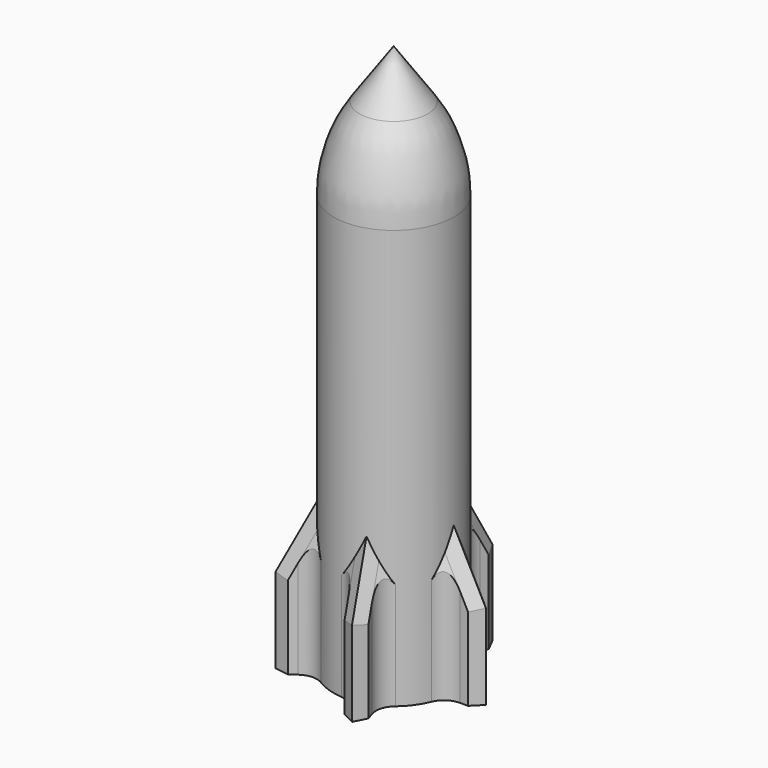
from build123d import *

# Parameters (mm, degrees)
F0_R          = 15.31
F0_R_2        = 11.5
F1_DEPTH      = 101.6
F2_DEPTH      = 25.4
F3_DEPTH      = 25.4
F4_DEPTH      = 25.4
F5_DEPTH      = 25.4
F6_R          = 15.31
F7_DEPTH      = 25.4
F7_TAPER      = 35
F8_T          = 2.54
F10_DEPTH     = 2.54
F11_DEPTH     = 10.668
F12_COUNT     = 5
F14_SIZE      = 2.5399
F15_DEPTH     = 25.4
F16_T1_DEPTH  = 31.2479879022
F16_T3_DEPTH  = 26.3887057153
F16_T5_DEPTH  = 18.1838383234
F16_T7_DEPTH  = 38.4641495789
F17_DEPTH     = 19.304
F18_R         = 36.6377921473
F19_T1_DEPTH  = 6.096
F19_T6_DEPTH  = 35.9639195383
F19_T11_DEPTH = 35.9639195383
F19_T16_DEPTH = 35.9639195383
F19_T21_DEPTH = 35.9639195383
F19_T26_DEPTH = 35.9639195383
F19_T31_DEPTH = 35.9639195383
F19_T36_DEPTH = 35.9639195383
F19_T41_DEPTH = 35.9639195383
F19_T46_DEPTH = 35.9639195383
F19_T51_DEPTH = 35.9639195383


# Not quite as in the source:
# - a fillet or chamfer that OpenCascade refuses, or shapes differently, is made with other operations: its cross-section is extruded or revolved along the edge and cut away or added
# - a fillet or chamfer is up to 0.001 mm smaller than in the source, because OpenCascade refuses the exact size
# - a shell that OpenCascade refuses in one call is made with other operations: the cavity is built on its own and cut out


with BuildPart() as f1:
    # F0 (on Top) → F1 (new body)
    with BuildSketch(Plane.XY):
        Circle(F0_R)
        Circle(F0_R_2, mode=Mode.SUBTRACT)
    extrude(amount=F1_DEPTH)

    # F2 (add): a face of the model
    f2_faces = [f1.faces().sort_by_distance(p)[0] for p in [
        (-14.8769678072, 0, 101.6),
    ]]
    extrude(f2_faces, amount=F2_DEPTH)

    # F3 (cut): a face of the model
    f3_faces = [f1.faces().sort_by_distance(p)[0] for p in [
        (-14.8769678072, 0, 127),
    ]]
    extrude(f3_faces, amount=-F3_DEPTH, mode=Mode.SUBTRACT)

    # F4 (add): a face of the model
    f4_faces = [f1.faces().sort_by_distance(p)[0] for p in [
        (-14.8769678072, 0, 101.6),
    ]]
    extrude(f4_faces, amount=F4_DEPTH)

    # F5 (cut): a face of the model
    f5_faces = [f1.faces().sort_by_distance(p)[0] for p in [
        (-14.8769678072, 0, 127),
    ]]
    extrude(f5_faces, amount=-F5_DEPTH, mode=Mode.SUBTRACT)

    # F6 (on face) → F7 (join)
    with BuildSketch(Plane.XY.offset(101.6)):
        Circle(F6_R)
    extrude(amount=F7_DEPTH, taper=F7_TAPER)

    # F8: shell of thickness 2.54, made by hand


with BuildPart() as f8_core1:
    # F8_t2: copy of F1
    add(f1.part)

    # the walls: a layer under each face that stays
    f8_faces = [f8_core1.faces().sort_by_distance(p)[0] for p in [
        (-15.31, 0, 50.8),
        (-7.655, 0, 112.5324729916),
        (-10.2066666667, -10.2066666667, 0),
        (-11.5, 0, 50.8),
    ]]
    thicken(f8_faces, amount=-F8_T, mode=Mode.SUBTRACT)


with BuildPart() as f1_1:
    add(f1.part)

    # what is left inside the walls is the cavity
    f8_cavity = [f8_core1.part.solids().sort_by_distance(p)[0] for p in [
        (-8.118682, 0, 107.397628),
    ]]
    add(f8_cavity, mode=Mode.SUBTRACT)

    # F9 (on Front) → F10 (join, symmetric)
    with BuildSketch(Plane.XZ):
        Polygon((26.068892777, 0), (12.5377972627, 26.279142328), (12.7, 0), align=None)
    extrude(amount=F10_DEPTH, both=True)

    # F11 (add): a face of the model
    f11_faces = [f1_1.faces().sort_by_distance(p)[0] for p in [
        (-14.7952381942, 0, 0),
    ]]
    extrude(f11_faces, amount=F11_DEPTH)


with BuildPart() as f12_1:
    # F12: instance of F1
    add(f1_1.part.rotate(Axis((0, 0, 0), (0, 0, 1)), 1 * 360 / F12_COUNT))


with BuildPart() as f12_2:
    # F12: instance of F1
    add(f1_1.part.rotate(Axis((0, 0, 0), (0, 0, 1)), 2 * 360 / F12_COUNT))


with BuildPart() as f12_3:
    # F12: instance of F1
    add(f1_1.part.rotate(Axis((0, 0, 0), (0, 0, 1)), 3 * 360 / F12_COUNT))


with BuildPart() as f12_4:
    # F12: instance of F1
    add(f1_1.part.rotate(Axis((0, 0, 0), (0, 0, 1)), 4 * 360 / F12_COUNT))


with BuildPart() as f12_2_1:
    add(f12_2.part)

    # F13: union F12_1, F1, F12_4, F12_3
    add(f12_1.part)
    add(f1_1.part)
    add(f12_4.part)
    add(f12_3.part)

    # F14 (size 2.54 in the source; OpenCascade refuses exactly that, so slightly less here)
    f14_edges = [f12_2_1.edges().sort_by_distance(p)[0] for p in [
        (20.583362, 2.54, 10.653612),
        (20.583362, -2.54, 10.653612),
        (8.776292, 18.791037, 10.653612),
        (3.944925, 20.360844, 10.653612),
        (-15.159315, 14.1535, 10.653612),
        (-18.145264, 10.043693, 10.653612),
        (-18.145264, -10.043693, 10.653612),
        (-15.159315, -14.1535, 10.653612),
        (8.776292, -18.791037, 10.653612),
        (3.944925, -20.360844, 10.653612),
    ]]
    chamfer(f14_edges, length=F14_SIZE)

    # F15 (add): a face of the model
    f15_faces = [f12_2_1.faces().sort_by_distance(p)[0] for p in [
        (-4.5128934655, 13.8892579239, -10.668),
    ]]
    extrude(f15_faces, amount=F15_DEPTH)

    # F16: chamfer of 5.08 on 13 edges, made by hand

    # F16_s2 → F16_t1 (cut)
    with BuildSketch(Plane.XY.offset(-23.7321495789)):
        Polygon((-15.4873964089, 14.391864802), (-22.583151822, 13.2680075522), (-19.5972027403, 17.3778138836), align=None)
        Polygon((-18.4733454905, 10.2820584706), (-19.5972027403, 17.3778138836), (-22.583151822, 13.2680075522), align=None)
        Polygon((-15.4873964089, -14.391864802), (-22.583151822, -13.2680075522), (-19.5972027403, -17.3778138836), align=None)
        Polygon((-18.4733454905, -10.2820584706), (-19.5972027403, -17.3778138836), (-22.583151822, -13.2680075522), align=None)
        Polygon((8.9016081126, -19.1767200797), (5.6400473412, -25.5778935139), (10.471414444, -24.0080871825), align=None)
        Polygon((4.0702410098, -20.7465264111), (10.471414444, -24.0080871825), (5.6400473412, -25.5778935139), align=None)
        Polygon((4.0702410098, 20.7465264111), (10.471414444, 24.0080871825), (5.6400473412, 25.5778935139), align=None)
        Polygon((8.9016081126, 19.1767200797), (5.6400473412, 25.5778935139), (10.471414444, 24.0080871825), align=None)
    extrude(amount=F16_T1_DEPTH, mode=Mode.SUBTRACT)

    # F16_s4 → F16_t3 (cut)
    with BuildSketch(Plane.XZ.offset(-13.1943528576)):
        Polygon((23.7433758033, 4.5164555577), (26.068892777, -5.08), (26.068892777, 0), align=None)
    extrude(amount=F16_T3_DEPTH, mode=Mode.SUBTRACT)

    # F16_s6 → F16_t5 (cut)
    with BuildSketch(Plane.XY.offset(-10.668)):
        Polygon((20.988892777, -2.54), (26.068892777, 2.54), (26.068892777, -2.54), align=None)
        Polygon((20.988892777, 2.54), (26.068892777, -2.54), (26.068892777, 2.54), align=None)
    extrude(amount=F16_T5_DEPTH, mode=Mode.SUBTRACT)

    # F16_s8 → F16_t7 (cut)
    with BuildSketch(Plane.XY.offset(-49.1321495789)):
        Polygon((20.988892777, -2.54), (26.068892777, 2.54), (26.068892777, -2.54), align=None)
        Polygon((20.988892777, 2.54), (26.068892777, -2.54), (26.068892777, 2.54), align=None)
    extrude(amount=F16_T7_DEPTH, mode=Mode.SUBTRACT)

    # F17 (cut): a face of the model
    f17_faces = [f12_2_1.faces().sort_by_distance(p)[0] for p in [
        (4.599928622, 20.1480200473, -36.068),
    ]]
    extrude(f17_faces, amount=-F17_DEPTH, mode=Mode.SUBTRACT)

    # F18
    f18_edges = [f12_2_1.edges().sort_by_distance(p)[0] for p in [
        (12.38605, -8.998992, 101.6),
    ]]
    fillet(f18_edges, radius=F18_R)

    # F19: fillet of radius 5.08 on 27 edges, made by hand

    # F19_s2 → F19_t1 (join)
    with BuildSketch(Plane.XY.offset(-16.764)):
        with BuildLine():
            ThreePointArc((14.2007070375, 5.7215399706), (16.0699037533, 3.4098588533), (18.9126333439, 2.54))
            Line((18.9126333439, 2.54), (15.09783097, 2.54))
            ThreePointArc((15.09783097, 2.54), (14.7353870492, 4.1550533702), (14.2007070375, 5.7215399706))
        make_face()
        with BuildLine():
            ThreePointArc((14.2007070375, -5.7215399706), (16.0699037533, -3.4098588533), (18.9126333439, -2.54))
            Line((18.9126333439, -2.54), (15.09783097, -2.54))
            ThreePointArc((15.09783097, -2.54), (14.7353870492, -4.1550533702), (14.2007070375, -5.7215399706))
        make_face()
        with BuildLine():
            ThreePointArc((-8.1255765104, 12.975789239), (-10.996560488, 12.2042861927), (-13.8076672428, 13.1714701273))
            Line((-13.8076672428, 13.1714701273), (-10.7214272921, 10.9291855515))
            ThreePointArc((-10.7214272921, 10.9291855515), (-9.4788994481, 12.0227519834), (-8.1255765104, 12.975789239))
        make_face()
        with BuildLine():
            ThreePointArc((-1.0532480655, 15.2737280489), (1.7229048756, 16.3370910149), (3.4286415603, 18.7718863477))
            Line((3.4286415603, 18.7718863477), (2.2498027966, 15.1437936917))
            ThreePointArc((2.2498027966, 15.1437936917), (0.6017944337, 15.2981679772), (-1.0532480655, 15.2737280489))
        make_face()
        with BuildLine():
            ThreePointArc((-14.8516501406, -3.7181430986), (-15.0050899808, -6.6870186712), (-16.7936163244, -9.0616637958))
            Line((-16.7936163244, -9.0616637958), (-13.7073763738, -6.8193792201))
            ThreePointArc((-13.7073763738, -6.8193792201), (-14.363457635, -5.2997344054), (-14.8516501406, -3.7181430986))
        make_face()
        with BuildLine():
            ThreePointArc((-14.8516501406, 3.7181430986), (-15.0050899808, 6.6870186712), (-16.7936163244, 9.0616637958))
            Line((-16.7936163244, 9.0616637958), (-13.7073763738, 6.8193792201))
            ThreePointArc((-13.7073763738, 6.8193792201), (-14.363457635, 5.2997344054), (-14.8516501406, 3.7181430986))
        make_face()
        with BuildLine():
            ThreePointArc((9.829767679, 11.7376218791), (8.2088418399, 14.2296823467), (8.260008663, 17.2020800163))
            Line((8.260008663, 17.2020800163), (7.0811698993, 13.5739873603))
            ThreePointArc((7.0811698993, 13.5739873603), (8.5051756002, 12.7302037694), (9.829767679, 11.7376218791))
        make_face()
        with BuildLine():
            ThreePointArc((-1.0532480655, -15.2737280489), (1.7229048756, -16.3370910149), (3.4286415603, -18.7718863477))
            Line((3.4286415603, -18.7718863477), (2.2498027966, -15.1437936917))
            ThreePointArc((2.2498027966, -15.1437936917), (0.6017944337, -15.2981679772), (-1.0532480655, -15.2737280489))
        make_face()
        with BuildLine():
            ThreePointArc((-8.1255765104, -12.975789239), (-10.996560488, -12.2042861927), (-13.8076672428, -13.1714701273))
            Line((-13.8076672428, -13.1714701273), (-10.7214272921, -10.9291855515))
            ThreePointArc((-10.7214272921, -10.9291855515), (-9.4788994481, -12.0227519834), (-8.1255765104, -12.975789239))
        make_face()
        with BuildLine():
            ThreePointArc((9.829767679, -11.7376218791), (8.2088418399, -14.2296823467), (8.260008663, -17.2020800163))
            Line((8.260008663, -17.2020800163), (7.0811698993, -13.5739873603))
            ThreePointArc((7.0811698993, -13.5739873603), (8.5051756002, -12.7302037694), (9.829767679, -11.7376218791))
        make_face()
    extrude(amount=F19_T1_DEPTH)


with BuildPart() as f19_tool4:
    # F19_s5 → F19_t6 (new body)
    with BuildSketch(Plane.XY.offset(-10.668)):
        with BuildLine():
            ThreePointArc((-8.1255765104, 12.975789239), (-10.996560488, 12.2042861927), (-13.8076672428, 13.1714701273))
            Line((-13.8076672428, 13.1714701273), (-10.7214272921, 10.9291855515))
            ThreePointArc((-10.7214272921, 10.9291855515), (-9.4788994481, 12.0227519834), (-8.1255765104, 12.975789239))
        make_face()
    extrude(amount=F19_T6_DEPTH)

    split(bisect_by=Plane(origin=(-1.5237102008, 15.4312558291, 5.3049866361), x_dir=(0.9951603879, 0.0982639424, 0), z_dir=(0.0929734367, -0.9415812046, -0.323698587)), keep=Keep.TOP)


with BuildPart() as f12_2_2:
    add(f12_2_1.part)

    # F19_t3: union F19_tool4
    add(f19_tool4.part)


with BuildPart() as f19_tool9:
    # F19_s10 → F19_t11 (new body)
    with BuildSketch(Plane.XY.offset(25.2959195383)):
        with BuildLine():
            ThreePointArc((-14.8516501406, 3.7181430986), (-15.0050899808, 6.6870186712), (-16.7936163244, 9.0616637958))
            Line((-16.7936163244, 9.0616637958), (-13.7073763738, 6.8193792201))
            ThreePointArc((-13.7073763738, 6.8193792201), (-14.363457635, 5.2997344054), (-14.8516501406, 3.7181430986))
        make_face()
    extrude(amount=-F19_T11_DEPTH)

    split(bisect_by=Plane(origin=(-15.1468487575, -3.3193857803, 5.3049866361), x_dir=(-0.2140669092, 0.9768189998, 0), z_dir=(0.9242273122, 0.202541601, -0.323698587)), keep=Keep.TOP)


with BuildPart() as f12_2_3:
    add(f12_2_2.part)

    # F19_t8: union F19_tool9
    add(f19_tool9.part)


with BuildPart() as f19_tool14:
    # F19_s15 → F19_t16 (new body)
    with BuildSketch(Plane.XY.offset(25.2959195383)):
        with BuildLine():
            ThreePointArc((-1.0532480655, 15.2737280489), (1.7229048756, 16.3370910149), (3.4286415603, 18.7718863477))
            Line((3.4286415603, 18.7718863477), (2.2498027966, 15.1437936917))
            ThreePointArc((2.2498027966, 15.1437936917), (0.6017944337, 15.2981679772), (-1.0532480655, 15.2737280489))
        make_face()
    extrude(amount=-F19_T16_DEPTH)

    split(bisect_by=Plane(origin=(-7.8375571537, 13.3797625951, 5.3049866361), x_dir=(0.8628597621, 0.5054434003, 0), z_dir=(0.4782304556, -0.816403611, -0.323698587)), keep=Keep.TOP)


with BuildPart() as f12_2_4:
    add(f12_2_3.part)

    # F19_t13: union F19_tool14
    add(f19_tool14.part)


with BuildPart() as f19_tool19:
    # F19_s20 → F19_t21 (new body)
    with BuildSketch(Plane.XY.offset(-10.668)):
        with BuildLine():
            ThreePointArc((-14.8516501406, -3.7181430986), (-15.0050899808, -6.6870186712), (-16.7936163244, -9.0616637958))
            Line((-16.7936163244, -9.0616637958), (-13.7073763738, -6.8193792201))
            ThreePointArc((-13.7073763738, -6.8193792201), (-14.363457635, -5.2997344054), (-14.8516501406, -3.7181430986))
        make_face()
    extrude(amount=F19_T21_DEPTH)

    split(bisect_by=Plane(origin=(-15.1468487575, 3.3193857803, 5.3049866361), x_dir=(0.2140669092, 0.9768189998, 0), z_dir=(0.9242273122, -0.202541601, -0.323698587)), keep=Keep.TOP)


with BuildPart() as f12_2_5:
    add(f12_2_4.part)

    # F19_t18: union F19_tool19
    add(f19_tool19.part)


with BuildPart() as f19_tool24:
    # F19_s25 → F19_t26 (new body)
    with BuildSketch(Plane.XY.offset(-10.668)):
        with BuildLine():
            ThreePointArc((9.829767679, 11.7376218791), (8.2088418399, 14.2296823467), (8.260008663, 17.2020800163))
            Line((8.260008663, 17.2020800163), (7.0811698993, 13.5739873603))
            ThreePointArc((7.0811698993, 13.5739873603), (8.5051756002, 12.7302037694), (9.829767679, 11.7376218791))
        make_face()
    extrude(amount=F19_T26_DEPTH)

    split(bisect_by=Plane(origin=(14.2051440643, 6.2176548112, 5.3049866361), x_dir=(0.4009760348, -0.9160885435, 0), z_dir=(-0.8667665683, -0.3793875866, -0.323698587)), keep=Keep.TOP)


with BuildPart() as f12_2_6:
    add(f12_2_5.part)

    # F19_t23: union F19_tool24
    add(f19_tool24.part)


with BuildPart() as f19_tool29:
    # F19_s30 → F19_t31 (new body)
    with BuildSketch(Plane.XY.offset(25.2959195383)):
        with BuildLine():
            ThreePointArc((-8.1255765104, -12.975789239), (-10.996560488, -12.2042861927), (-13.8076672428, -13.1714701273))
            Line((-13.8076672428, -13.1714701273), (-10.7214272921, -10.9291855515))
            ThreePointArc((-10.7214272921, -10.9291855515), (-9.4788994481, -12.0227519834), (-8.1255765104, -12.975789239))
        make_face()
    extrude(amount=-F19_T31_DEPTH)

    split(bisect_by=Plane(origin=(-1.5237102008, -15.4312558291, 5.3049866361), x_dir=(-0.9951603879, 0.0982639424, 0), z_dir=(0.0929734367, 0.9415812046, -0.323698587)), keep=Keep.TOP)


with BuildPart() as f12_2_7:
    add(f12_2_6.part)

    # F19_t28: union F19_tool29
    add(f19_tool29.part)


with BuildPart() as f19_tool34:
    # F19_s35 → F19_t36 (new body)
    with BuildSketch(Plane.XY.offset(25.2959195383)):
        with BuildLine():
            ThreePointArc((14.2007070375, 5.7215399706), (16.0699037533, 3.4098588533), (18.9126333439, 2.54))
            Line((18.9126333439, 2.54), (15.09783097, 2.54))
            ThreePointArc((15.09783097, 2.54), (14.7353870492, 4.1550533702), (14.2007070375, 5.7215399706))
        make_face()
    extrude(amount=-F19_T36_DEPTH)

    split(bisect_by=Plane(origin=(10.3029720477, 11.5885338255, 5.3049866361), x_dir=(0.7473435697, -0.664437799, 0), z_dir=(-0.6286646362, -0.7071067812, -0.323698587)), keep=Keep.TOP)


with BuildPart() as f12_2_8:
    add(f12_2_7.part)

    # F19_t33: union F19_tool34
    add(f19_tool34.part)


with BuildPart() as f19_tool39:
    # F19_s40 → F19_t41 (new body)
    with BuildSketch(Plane.XY.offset(-10.668)):
        with BuildLine():
            ThreePointArc((-1.0532480655, -15.2737280489), (1.7229048756, -16.3370910149), (3.4286415603, -18.7718863477))
            Line((3.4286415603, -18.7718863477), (2.2498027966, -15.1437936917))
            ThreePointArc((2.2498027966, -15.1437936917), (0.6017944337, -15.2981679772), (-1.0532480655, -15.2737280489))
        make_face()
    extrude(amount=F19_T41_DEPTH)

    split(bisect_by=Plane(origin=(-7.8375571537, -13.3797625951, 5.3049866361), x_dir=(-0.8628597621, 0.5054434003, 0), z_dir=(0.4782304556, 0.816403611, -0.323698587)), keep=Keep.TOP)


with BuildPart() as f12_2_9:
    add(f12_2_8.part)

    # F19_t38: union F19_tool39
    add(f19_tool39.part)


with BuildPart() as f19_tool44:
    # F19_s45 → F19_t46 (new body)
    with BuildSketch(Plane.XY.offset(-10.668)):
        with BuildLine():
            ThreePointArc((14.2007070375, -5.7215399706), (16.0699037533, -3.4098588533), (18.9126333439, -2.54))
            Line((18.9126333439, -2.54), (15.09783097, -2.54))
            ThreePointArc((15.09783097, -2.54), (14.7353870492, -4.1550533702), (14.2007070375, -5.7215399706))
        make_face()
    extrude(amount=F19_T46_DEPTH)

    split(bisect_by=Plane(origin=(10.3029720477, -11.5885338255, 5.3049866361), x_dir=(-0.7473435697, -0.664437799, 0), z_dir=(-0.6286646362, 0.7071067812, -0.323698587)), keep=Keep.TOP)


with BuildPart() as f12_2_10:
    add(f12_2_9.part)

    # F19_t43: union F19_tool44
    add(f19_tool44.part)


with BuildPart() as f19_tool49:
    # F19_s50 → F19_t51 (new body)
    with BuildSketch(Plane.XY.offset(25.2959195383)):
        with BuildLine():
            ThreePointArc((9.829767679, -11.7376218791), (8.2088418399, -14.2296823467), (8.260008663, -17.2020800163))
            Line((8.260008663, -17.2020800163), (7.0811698993, -13.5739873603))
            ThreePointArc((7.0811698993, -13.5739873603), (8.5051756002, -12.7302037694), (9.829767679, -11.7376218791))
        make_face()
    extrude(amount=-F19_T51_DEPTH)

    split(bisect_by=Plane(origin=(14.2051440643, -6.2176548112, 5.3049866361), x_dir=(-0.4009760348, -0.9160885435, 0), z_dir=(-0.8667665683, 0.3793875866, -0.323698587)), keep=Keep.TOP)


with BuildPart() as f12_2_11:
    add(f12_2_10.part)

    # F19_t48: union F19_tool49
    add(f19_tool49.part)


solid = f12_2_11.part
